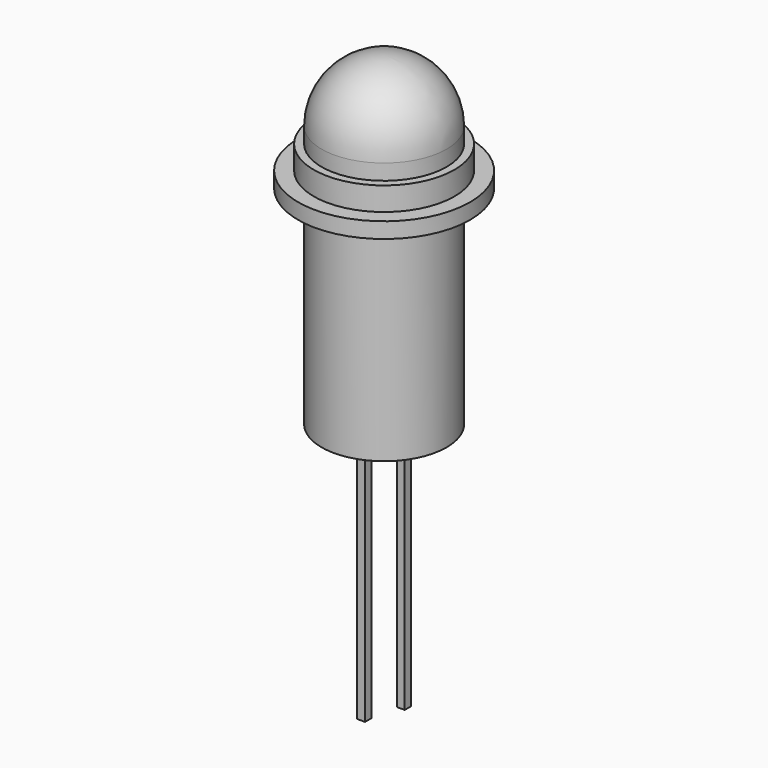
from build123d import *

# Parameters (mm, degrees)
F0_R      = 5.5
F1_DEPTH  = 1
F2_R      = 4.5
F3_DEPTH  = 1.5
F4_R      = 4
F5_DEPTH  = 5
F6_R      = 4
F7_R      = 4
F8_DEPTH  = 13.3
F9_W      = 0.5
F9_H      = 0.5
F10_DEPTH = 15.5
F11_W     = 0.5
F11_H     = 0.5
F12_DEPTH = 1.5


with BuildPart() as f1:
    # F0 (on Top) → F1 (new body)
    with BuildSketch(Plane.XY):
        Circle(F0_R)
    extrude(amount=F1_DEPTH)

    # F2 (on face) → F3 (join)
    with BuildSketch(Plane.XY.offset(1)):
        Circle(F2_R)
    extrude(amount=F3_DEPTH)

    # F4 (on face) → F5 (join)
    with BuildSketch(Plane.XY.offset(2.5)):
        Circle(F4_R)
    extrude(amount=F5_DEPTH)

    # F6
    f6_edges = [f1.edges().sort_by_distance(p)[0] for p in [
        (-4, 0, 7.5),
    ]]
    fillet(f6_edges, radius=F6_R)

    # F7 (on face) → F8 (join)
    with BuildSketch(Plane(origin=(0, 0, 0), x_dir=(1, 0, 0), z_dir=(0, 0, -1))):
        Circle(F7_R)
    extrude(amount=F8_DEPTH)

    # F9 (on face) → F10 (join)
    with BuildSketch(Plane(origin=(0, 0, -13.3), x_dir=(1, 0, 0), z_dir=(0, 0, -1))):
        with Locations((-1.27, 0)):
            Rectangle(F9_W, F9_H)
        with Locations((1.27, 0)):
            Rectangle(F9_W, F9_H)
    extrude(amount=F10_DEPTH)

    # F11 (on face) → F12 (join)
    with BuildSketch(Plane(origin=(0, 0, -28.8), x_dir=(1, 0, 0), z_dir=(0, 0, -1))):
        with Locations((-1.27, 0)):
            Rectangle(F11_W, F11_H)
    extrude(amount=F12_DEPTH)


solid = f1.part
